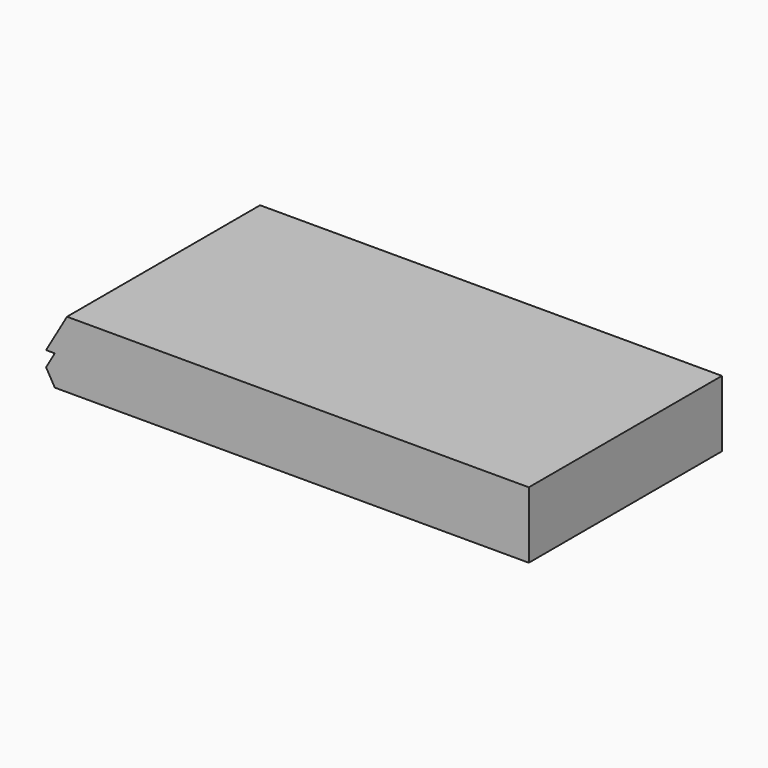
from build123d import *

# Parameters (mm, degrees)
F0_W     = 254
F0_H     = 127
F1_DEPTH = 15.9
F3_DEPTH = 127
F4_W     = 4.5899346401
F4_H     = 127
F4_W_2   = 249.4100653599
F5_DEPTH = 19.05
F7_DEPTH = 127


# Not quite as in the source:
# - the program builds the solid bodies; features that only make, move or delete a surface that nothing else refers to are left out


with BuildPart() as f1:
    # F0 (on Top) → F1 (new body)
    with BuildSketch(Plane.XY):
        with Locations((10.4389302433, -20.9855538282)):
            Rectangle(F0_W, F0_H)
    extrude(amount=-F1_DEPTH)

    # F2 (on face) → F3 (cut)
    with BuildSketch(Plane.XZ.offset(84.4855538282)):
        Polygon((-116.5610697567, 0), (-116.5610697567, -7.95), (-111.9711351167, 0), align=None)
        Polygon((-111.9711351167, -15.9), (-116.5610697567, -7.95), (-116.5610697567, -15.9), align=None)
    extrude(amount=-F3_DEPTH, mode=Mode.SUBTRACT)

    # F4 (on face) → F5 (join)
    with BuildSketch(Plane.XY):
        with Locations((-114.2661024367, -20.9855538282)):
            Rectangle(F4_W, F4_H)
        with Locations((12.7338975633, -20.9855538282)):
            Rectangle(F4_W_2, F4_H)
    extrude(amount=F5_DEPTH)

    # F6 (on face) → F7 (cut)
    with BuildSketch(Plane.XZ.offset(84.4855538282)):
        Polygon((-116.5610697567, 19.05), (-116.5610697567, 0), (-105.5625471287, 19.05), align=None)
    extrude(amount=-F7_DEPTH, mode=Mode.SUBTRACT)


solid = f1.part
